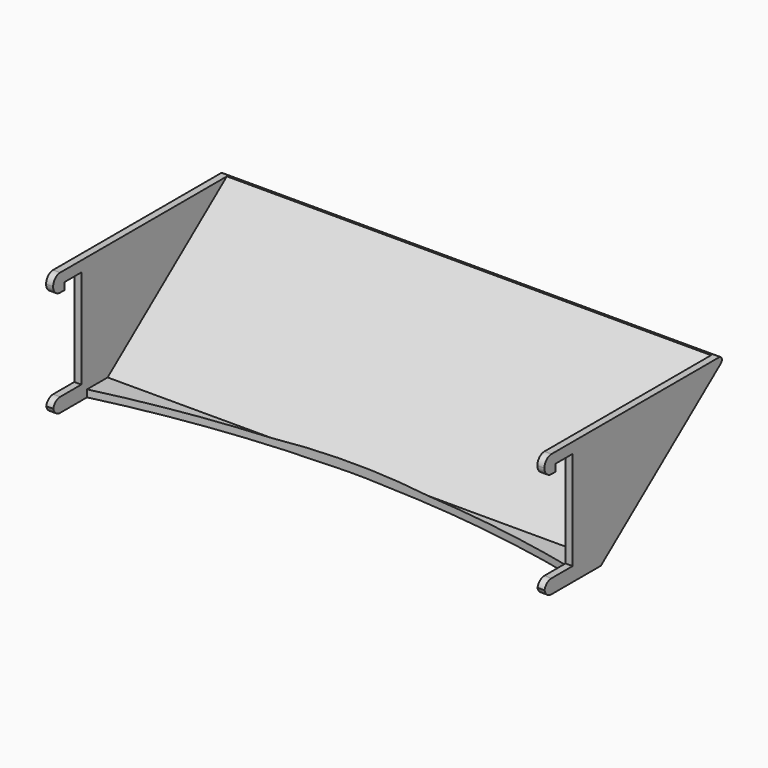
from build123d import *

# Parameters (mm, degrees)
F1_DEPTH     = 89.69375
F2_DEPTH     = 12.7
F4_DEPTH     = 44.451
F5_T         = 2.54
F6_R         = 1.27
F7_W         = 2.54
F7_H         = 3.81
F7_H_2       = 5.08
F8_W         = 2.54
F8_H         = 3.81
F8_H_2       = 5.08
F9_DEPTH     = 12.7
F11_W        = 2.54
F11_H        = 5.08
F10_W        = 2.54
F10_H        = 5.08
F12_DEPTH    = 2.54
F13_T1_DEPTH = 18.415
F13_T3_DEPTH = 18.415


# Not quite as in the source:
# - a fillet or chamfer that OpenCascade refuses, or shapes differently, is made with other operations: its cross-section is extruded or revolved along the edge and cut away or added
# - a shell that OpenCascade refuses in one call is made with other operations: the cavity is built on its own and cut out
# - a feature names something its author has since deleted; it is built from what else it names


with BuildPart() as f1:
    # F0 (on Right) → F1 (new body, symmetric)
    with BuildSketch(Plane.YZ):
        Polygon((0, 44.45), (0, 0), (56.893405551, 44.45), align=None)
    extrude(amount=F1_DEPTH, both=True)

    # F2 (add): a face of the model
    f2_faces = [f1.faces().sort_by_distance(p)[0] for p in [
        (0, 0, 22.225),
    ]]
    extrude(f2_faces, amount=F2_DEPTH)

    # F3 (on face) → F4 (cut, through all)
    with BuildSketch(Plane.XY.offset(44.45)):
        with BuildLine():
            Line((-87.15375, -10.16), (-87.15375, -12.7))
            Line((-87.15375, -12.7), (87.15375, -12.7))
            Line((87.15375, -12.7), (87.15375, -10.16))
            ThreePointArc((87.15375, -10.16), (0, 0.1903063345), (-87.15375, -10.16))
        make_face()
    extrude(amount=-F4_DEPTH, mode=Mode.SUBTRACT)

    # F5: shell of thickness 2.54, made by hand


with BuildPart() as f5_core1:
    # F5_t2: copy of F1
    add(f1.part)

    # the walls: a layer under each face that stays
    f5_faces = [f5_core1.faces().sort_by_distance(p)[0] for p in [
        (0, 28.4467027755, 22.225),
        (89.69375, 22.0967027755, 22.225),
        (88.42375, -12.7, 22.225),
        (87.15375, -11.43, 22.225),
        (-87.15375, -11.43, 22.225),
        (-88.42375, -12.7, 22.225),
        (-89.69375, 22.0967027755, 22.225),
        (-76.7280098971, -6.35, 0),
        (50.7965296912, -2.1166666667, 0),
    ]]
    thicken(f5_faces, amount=-F5_T, mode=Mode.SUBTRACT)


with BuildPart() as f1_1:
    add(f1.part)

    # what is left inside the walls is the cavity
    f5_cavity = [f5_core1.part.solids().sort_by_distance(p)[0] for p in [
        (-29.05125, 25.930947, 23.515015),
    ]]
    add(f5_cavity, mode=Mode.SUBTRACT)

    # F6
    f6_edges = [f1_1.edges().sort_by_distance(p)[0] for p in [
        (0, 56.893406, 44.45),
    ]]
    fillet(f6_edges, radius=F6_R)

    # F7 (on face) + F8 (on face) → F9 (join)
    with BuildSketch(Plane.XZ.offset(12.7)):
        with Locations((-88.42375, 42.545)):
            Rectangle(F7_W, F7_H)
        with Locations((-88.42375, 2.54)):
            Rectangle(F7_W, F7_H_2)
    with BuildSketch(Plane.XZ.offset(12.7)):
        with Locations((88.42375, 42.545)):
            Rectangle(F8_W, F8_H)
        with Locations((88.42375, 2.54)):
            Rectangle(F8_W, F8_H_2)
    extrude(amount=F9_DEPTH)

    # F11 (on face) + F10 (on face) → F12 (join)
    with BuildSketch(Plane(origin=(0, 0, 40.64), x_dir=(1, 0, 0), z_dir=(0, 0, -1))):
        with Locations((-88.42375, 22.86)):
            Rectangle(F11_W, F11_H)
    with BuildSketch(Plane(origin=(0, 0, 40.64), x_dir=(1, 0, 0), z_dir=(0, 0, -1))):
        with Locations((88.42375, 22.86)):
            Rectangle(F10_W, F10_H)
    extrude(amount=F12_DEPTH)

    # F13: fillet of radius 3.175 on 8 edges, made by hand

    # F13_s2 → F13_t1 (cut)
    with BuildSketch(Plane.YZ.offset(79.21625)):
        with BuildLine():
            ThreePointArc((-22.225, 44.45), (-24.4700640303, 43.5200640303), (-25.4, 41.275))
            Line((-25.4, 41.275), (-25.4, 44.45))
            Line((-25.4, 44.45), (-22.225, 44.45))
        make_face()
        with BuildLine():
            ThreePointArc((-22.225, 38.1), (-24.4700640303, 39.0299359697), (-25.4, 41.275))
            Line((-25.4, 41.275), (-25.4, 38.1))
            Line((-25.4, 38.1), (-22.225, 38.1))
        make_face()
        with BuildLine():
            ThreePointArc((-25.4, 1.905), (-24.4700640303, 4.1500640303), (-22.225, 5.08))
            Line((-22.225, 5.08), (-25.4, 5.08))
            Line((-25.4, 5.08), (-25.4, 1.905))
        make_face()
        with BuildLine():
            ThreePointArc((-22.225, 0), (-24.4700640303, 0.9299359697), (-25.4, 3.175))
            Line((-25.4, 3.175), (-25.4, 0))
            Line((-25.4, 0), (-22.225, 0))
        make_face()
    extrude(amount=F13_T1_DEPTH, mode=Mode.SUBTRACT)

    # F13_s4 → F13_t3 (cut)
    with BuildSketch(Plane.YZ.offset(-97.63125)):
        with BuildLine():
            ThreePointArc((-22.225, 44.45), (-24.4700640303, 43.5200640303), (-25.4, 41.275))
            Line((-25.4, 41.275), (-25.4, 44.45))
            Line((-25.4, 44.45), (-22.225, 44.45))
        make_face()
        with BuildLine():
            ThreePointArc((-22.225, 38.1), (-24.4700640303, 39.0299359697), (-25.4, 41.275))
            Line((-25.4, 41.275), (-25.4, 38.1))
            Line((-25.4, 38.1), (-22.225, 38.1))
        make_face()
        with BuildLine():
            ThreePointArc((-25.4, 1.905), (-24.4700640303, 4.1500640303), (-22.225, 5.08))
            Line((-22.225, 5.08), (-25.4, 5.08))
            Line((-25.4, 5.08), (-25.4, 1.905))
        make_face()
        with BuildLine():
            ThreePointArc((-22.225, 0), (-24.4700640303, 0.9299359697), (-25.4, 3.175))
            Line((-25.4, 3.175), (-25.4, 0))
            Line((-25.4, 0), (-22.225, 0))
        make_face()
    extrude(amount=F13_T3_DEPTH, mode=Mode.SUBTRACT)


solid = f1_1.part
